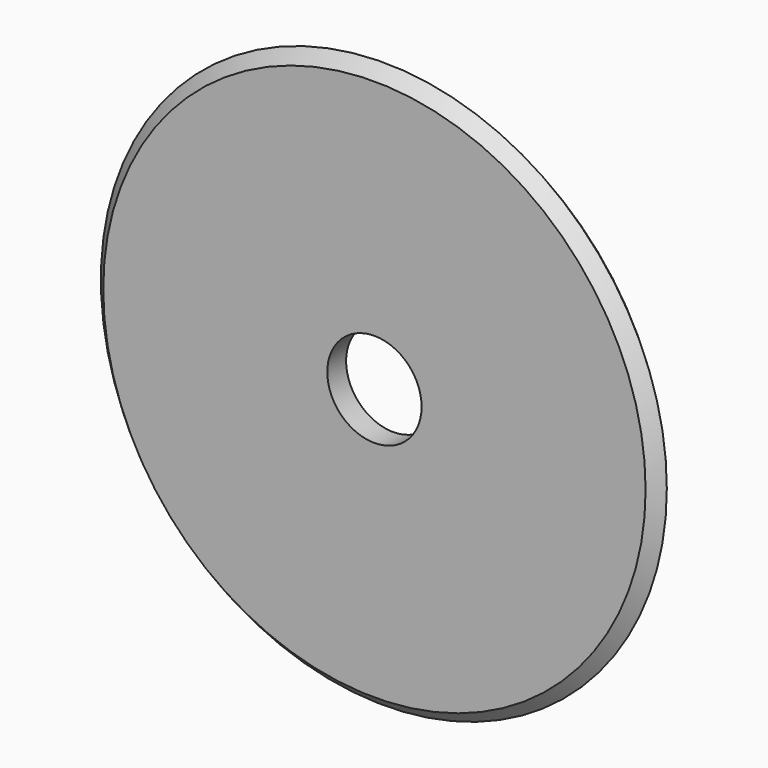
from build123d import *

# Parameters (mm, degrees)
F0_R     = 38.1
F0_R_2   = 6.35
F1_DEPTH = 1.5875
F2_SIZE  = 1.58749


# Not quite as in the source:
# - a fillet or chamfer is up to 0.001 mm smaller than in the source, because OpenCascade refuses the exact size


with BuildPart() as f1:
    # F0 (on Front) → F1 (new body, symmetric)
    with BuildSketch(Plane.XZ):
        Circle(F0_R)
        Circle(F0_R_2, mode=Mode.SUBTRACT)
    extrude(amount=F1_DEPTH, both=True)

    # F2 (size 1.5875 in the source; OpenCascade refuses exactly that, so slightly less here)
    f2_edges = [f1.edges().sort_by_distance(p)[0] for p in [
        (-38.1, 1.5875, 0),
        (-38.1, -1.5875, 0),
    ]]
    chamfer(f2_edges, length=F2_SIZE)


solid = f1.part
